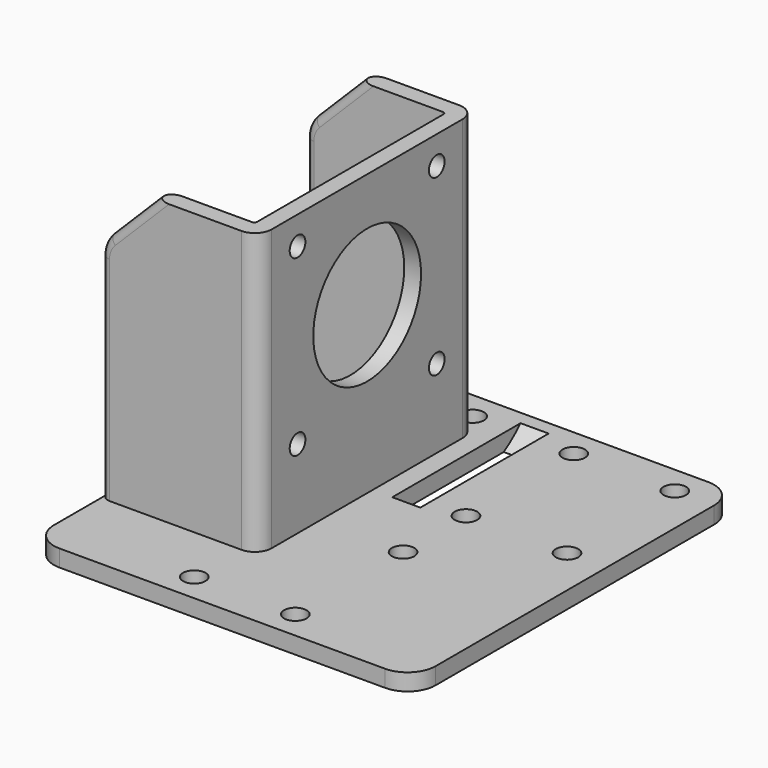
from build123d import *

# Parameters (mm, degrees)
F0_W      = 68
F0_H      = 72
F0_R      = 2
F1_DEPTH  = 3
F3_DEPTH  = 50
F4_SIZE   = 10
F6_R      = 1.75
F6_R_2    = 12
F7_DEPTH  = 25
F8_R      = 5
F9_R      = 1.49999
F10_R     = 3
F11_R     = 0.5
F13_R     = 20
F13_R_2   = 1.75
F14_DEPTH = 2.5


# Not quite as in the source:
# - a fillet or chamfer is up to 0.001 mm smaller than in the source, because OpenCascade refuses the exact size


with BuildPart() as f1:
    # F0 (on Top) → F1 (new body)
    with BuildSketch(Plane.XY):
        with Locations((0, 36)):
            Rectangle(F0_W, F0_H)
        with Locations((-9, 5)):
            Circle(F0_R, mode=Mode.SUBTRACT)
        with Locations((-9, 29)):
            Circle(F0_R, mode=Mode.SUBTRACT)
        with Locations((9, 5)):
            Circle(F0_R, mode=Mode.SUBTRACT)
        with Locations((9, 29)):
            Circle(F0_R, mode=Mode.SUBTRACT)
        with Locations((-27, 43)):
            Circle(F0_R, mode=Mode.SUBTRACT)
        with Locations((-9, 43)):
            Circle(F0_R, mode=Mode.SUBTRACT)
        with Locations((-27, 67)):
            Circle(F0_R, mode=Mode.SUBTRACT)
        with Locations((-9, 67)):
            Circle(F0_R, mode=Mode.SUBTRACT)
        with Locations((9, 43)):
            Circle(F0_R, mode=Mode.SUBTRACT)
        with Locations((27, 43)):
            Circle(F0_R, mode=Mode.SUBTRACT)
        with Locations((9, 67)):
            Circle(F0_R, mode=Mode.SUBTRACT)
        with Locations((27, 67)):
            Circle(F0_R, mode=Mode.SUBTRACT)
        with Locations((-9, 43)):
            Circle(F0_R)
        with Locations((-9, 29)):
            Circle(F0_R)
    extrude(amount=-F1_DEPTH)

    # F2 (on Top) → F3 (join)
    with BuildSketch(Plane.XY):
        Polygon((-6, 64), (-34, 64), (-34, 61), (-9, 61), (-9, 18.5), (-34, 18.5), (-34, 15.5), (-6, 15.5), align=None)
    extrude(amount=F3_DEPTH)

    # F4
    f4_edges = [f1.edges().sort_by_distance(p)[0] for p in [
        (-34, 62.5, 50),
        (-34, 17, 50),
    ]]
    chamfer(f4_edges, length=F4_SIZE)

    # F6 (on face) → F7 (cut)
    with BuildSketch(Plane.YZ.offset(-6)):
        with Locations((55.25, 45)):
            Circle(F6_R)
        with Locations((39.75, 29.5)):
            Circle(F6_R_2)
        with Locations((55.25, 14)):
            Circle(F6_R)
        with Locations((24.25, 45)):
            Circle(F6_R)
        with Locations((24.25, 14)):
            Circle(F6_R)
    extrude(amount=-F7_DEPTH, mode=Mode.SUBTRACT)

    # F8
    f8_edges = [f1.edges().sort_by_distance(p)[0] for p in [
        (-34, 72, -1.5),
        (34, 72, -1.5),
        (34, 0, -1.5),
        (-34, 0, -1.5),
        (-34, 17, 40),
        (-34, 62.5, 40),
    ]]
    fillet(f8_edges, radius=F8_R)

    # F9 (radius 1.5 in the source; OpenCascade refuses exactly that, so slightly less here)
    f9_edges = [f1.edges().sort_by_distance(p)[0] for p in [
        (-34, 64, 18.964466),
        (-34, 61, 18.964466),
        (-28.267767, 15.5, 45.732233),
        (-28.267767, 18.5, 45.732233),
        (-33.619398, 15.5, 39.842349),
        (-34, 15.5, 18.964466),
        (-34, 18.5, 18.964466),
        (-33.619398, 18.5, 39.842349),
        (-33.619398, 64, 39.842349),
        (-33.619398, 61, 39.842349),
        (-28.267767, 61, 45.732233),
        (-28.267767, 64, 45.732233),
    ]]
    fillet(f9_edges, radius=F9_R)

    # F10
    f10_edges = [f1.edges().sort_by_distance(p)[0] for p in [
        (-6, 15.5, 25),
        (-6, 64, 25),
    ]]
    fillet(f10_edges, radius=F10_R)

    # F11
    f11_edges = [f1.edges().sort_by_distance(p)[0] for p in [
        (-9, 18.5, 25),
        (-9, 61, 25),
    ]]
    fillet(f11_edges, radius=F11_R)

    # F13 (on offset) → F14 (cut, symmetric)
    with BuildSketch(Plane.YZ):
        with Locations((55.25, 14)):
            Circle(F13_R)
        with Locations((55.25, 14)):
            Circle(F13_R_2, mode=Mode.SUBTRACT)
    extrude(amount=F14_DEPTH, both=True, mode=Mode.SUBTRACT)


solid = f1.part
